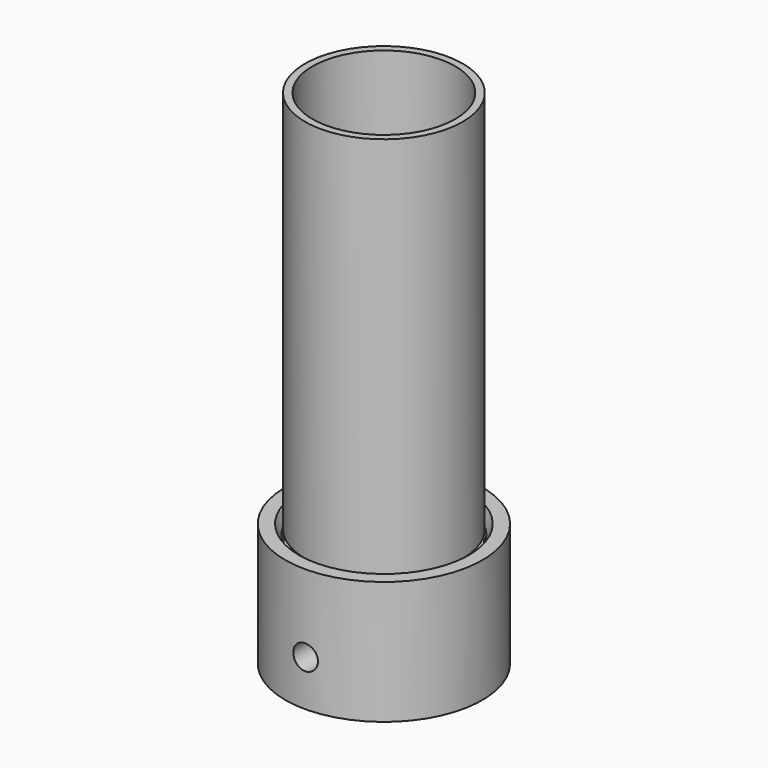
from build123d import *

# Parameters (mm, degrees)
F0_R           = 16
F0_R_2         = 14.5
F1_DEPTH       = 80
F6_D           = 3
F6_DEPTH       = 22
F6_CBORE_D     = 5
F6_CBORE_DEPTH = 5
F6_TIP         = 0.9012909285
F9_D           = 3
F9_DEPTH       = 22
F9_CBORE_D     = 5
F9_CBORE_DEPTH = 5
F9_TIP         = 0.9012909285
F11_R          = 15.9
F12_DEPTH      = 1
F13_R          = 1.5
F14_DEPTH      = 1
F15_R          = 14.5
F16_DEPTH      = 40
F18_R          = 15.9
F19_DEPTH      = 0.5
F21_SIZE2      = 1
F21_SIZE       = 2
F22_SIZE2      = 1.49999
F22_SIZE       = 1.99999


# Not quite as in the source:
# - a fillet or chamfer is up to 0.001 mm smaller than in the source, because OpenCascade refuses the exact size


with BuildPart() as f1:
    # F0 (on Top) → F1 (new body)
    with BuildSketch(Plane.XY):
        Circle(F0_R)
        Circle(F0_R_2, mode=Mode.SUBTRACT)
    extrude(amount=F1_DEPTH)


with BuildPart() as f3:
    # F2 (on Front) → F3 (revolve)
    with BuildSketch(Plane.XZ):
        Polygon((-14.1818207945, 0), (-16.25, 0), (-16.25, 5), (-20, 5), (-20, -20), (0, -20), (0, -12), (-14.1818207945, -3), align=None)
    revolve(axis=Axis((0, 0, -16), (0, 0, 1)))

    # F6
    with Locations(Plane.XZ.offset(20)):
        with Locations((0, -10.7207391411)):
            CounterBoreHole(F6_D / 2, F6_CBORE_D / 2, F6_CBORE_DEPTH, depth=F6_DEPTH)
            with Locations((0, 0, -(F6_DEPTH + F6_TIP / 2))):  # 118° drill point
                Cone(0, F6_D / 2, F6_TIP, mode=Mode.SUBTRACT)

    # F9
    with Locations(Plane(origin=(0, 20, 0), x_dir=(1, 0, 0), z_dir=(0, 1, 0))):
        with Locations((0, 5.594058428)):
            CounterBoreHole(F9_D / 2, F9_CBORE_D / 2, F9_CBORE_DEPTH, depth=F9_DEPTH)
            with Locations((0, 0, -(F9_DEPTH + F9_TIP / 2))):  # 118° drill point
                Cone(0, F9_D / 2, F9_TIP, mode=Mode.SUBTRACT)

    # F21
    f21_edges = [f3.edges().sort_by_distance(p)[0] for p in [
        (16.25, 0, 5),
    ]]
    f21_side = f3.faces().sort_by_distance((16.25, 0, 2.5))[0]
    chamfer(f21_edges, length=F21_SIZE, length2=F21_SIZE2, reference=f21_side)


with BuildPart() as f1_1:
    # F10: moved
    add(f1.part.moved(Location((0, 0, 2))))

    # F22 (size 2 and 1.5 in the source; OpenCascade refuses exactly that, so slightly less here)
    f22_edges = [f1_1.edges().sort_by_distance(p)[0] for p in [
        (-16, 0, 2),
    ]]
    f22_side = f1_1.faces().sort_by_distance((-16, 0, 42))[0]
    chamfer(f22_edges, length=F22_SIZE, length2=F22_SIZE2, reference=f22_side)


with BuildPart() as f12:
    # F11 (on Top) → F12 (new body)
    with BuildSketch(Plane.XY):
        Circle(F11_R)
    extrude(amount=F12_DEPTH)

    # F13 (on Top) → F14 (cut)
    with BuildSketch(Plane.XY):
        with Locations((6.4248272051, -8.8430160073)):
            Circle(F13_R)
        with Locations((-6.4248272051, -8.8430160073)):
            Circle(F13_R)
        with Locations((-10.3955887897, -3.3777315517)):
            Circle(F13_R)
        with Locations((0, -10.9305689111)):
            Circle(F13_R)
        with Locations((-6.4248272051, 8.8430160073)):
            Circle(F13_R)
        with Locations((3.3777315517, 10.3955887897)):
            Circle(F13_R)
        with Locations((-10.3955887897, 3.3777315517)):
            Circle(F13_R)
        with Locations((0, 10.9305689111)):
            Circle(F13_R)
        with Locations((-5.7666221108, 4.1896962064)):
            Circle(F13_R)
        with Locations((2.8609776839, 2.0786219591)):
            Circle(F13_R)
        with Locations((-5.7666221108, -4.1896962064)):
            Circle(F13_R)
        with Locations((-3.3777315517, 10.3955887897)):
            Circle(F13_R)
        with Locations((8.8430160073, -6.4248272051)):
            Circle(F13_R)
        with Locations((-3.5363628995, 0)):
            Circle(F13_R)
        with Locations((-2.202653646, -6.7790708645)):
            Circle(F13_R)
        with Locations((-2.202653646, 6.7790708645)):
            Circle(F13_R)
        with Locations((8.8430160073, 6.4248272051)):
            Circle(F13_R)
        with Locations((2.202653646, 6.7790708645)):
            Circle(F13_R)
        with Locations((6.4248272051, 8.8430160073)):
            Circle(F13_R)
        Circle(F13_R)
        with Locations((10.3955887897, -3.3777315517)):
            Circle(F13_R)
        with Locations((10.9305689111, 0)):
            Circle(F13_R)
        with Locations((5.7666221108, 4.1896962064)):
            Circle(F13_R)
        with Locations((5.7666221108, -4.1896962064)):
            Circle(F13_R)
        with Locations((10.3955887897, 3.3777315517)):
            Circle(F13_R)
        with Locations((2.202653646, -6.7790708645)):
            Circle(F13_R)
        with Locations((-7.1279369295, 0)):
            Circle(F13_R)
        with Locations((-1.0927962342, -3.3632809795)):
            Circle(F13_R)
        with Locations((3.3777315517, -10.3955887897)):
            Circle(F13_R)
        with Locations((2.8609776839, -2.0786219591)):
            Circle(F13_R)
        with Locations((-1.0927962342, 3.3632809795)):
            Circle(F13_R)
        with Locations((-3.3777315517, -10.3955887897)):
            Circle(F13_R)
        with Locations((-8.8430160073, -6.4248272051)):
            Circle(F13_R)
        with Locations((-10.9305689111, 0)):
            Circle(F13_R)
        with Locations((-8.8430160073, 6.4248272051)):
            Circle(F13_R)
        with Locations((7.1279369295, 0)):
            Circle(F13_R)
    extrude(amount=F14_DEPTH, mode=Mode.SUBTRACT)


with BuildPart() as f16:
    # F15 (on Top) → F16 (new body)
    with BuildSketch(Plane.XY):
        Circle(F15_R)
    extrude(amount=F16_DEPTH)


with BuildPart() as f16_1:
    # F17: moved
    add(f16.part.moved(Location((0, 0, 2))))


with BuildPart() as f19:
    # F18 (on Top) → F19 (new body)
    with BuildSketch(Plane.XY):
        Circle(F18_R)
    extrude(amount=F19_DEPTH)


with BuildPart() as f19_1:
    # F20: moved
    add(f19.part.moved(Location((0, 0, 1.25))))


with BuildPart() as f23_1:
    # F23: copy of F3
    add(f3.part)


solid = Compound([f1_1.part, f12.part, f16_1.part, f19_1.part, f23_1.part])
